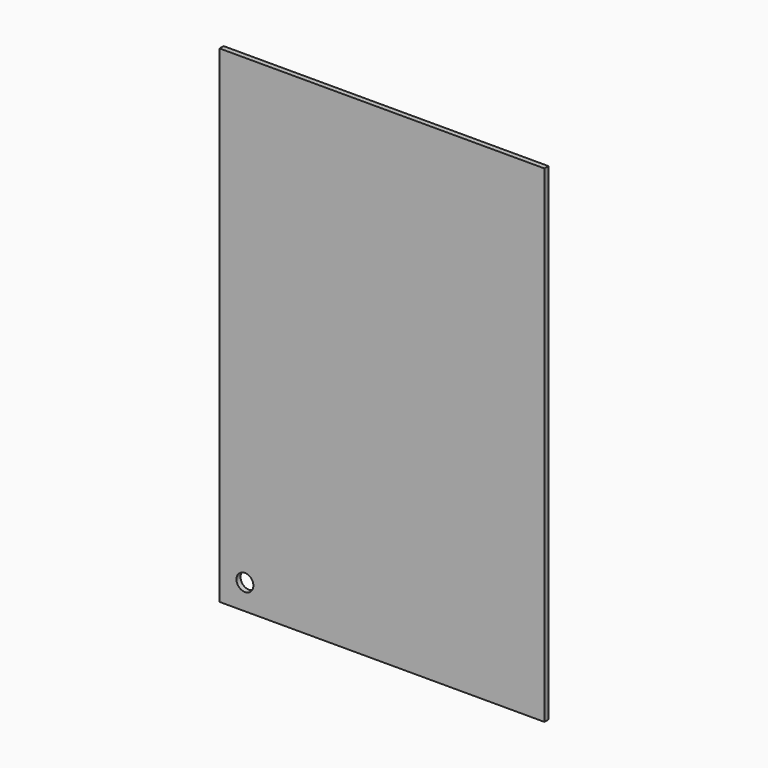
from build123d import *

# Parameters (mm, degrees)
F0_W     = 1219.2
F0_H     = 1828.8
F0_R     = 31.75
F1_DEPTH = 19.05


# Not quite as in the source:
# - the program builds the solid bodies; features that only make, move or delete a surface that nothing else refers to are left out


with BuildPart() as f1:
    # F0 (on Front) → F1 (new body)
    with BuildSketch(Plane.XZ):
        with Locations((-3.8652196527, 619.5944768926)):
            Rectangle(F0_W, F0_H)
        with Locations((-518.2152196527, -199.5555231074)):
            Circle(F0_R, mode=Mode.SUBTRACT)
    extrude(amount=F1_DEPTH)


solid = f1.part
